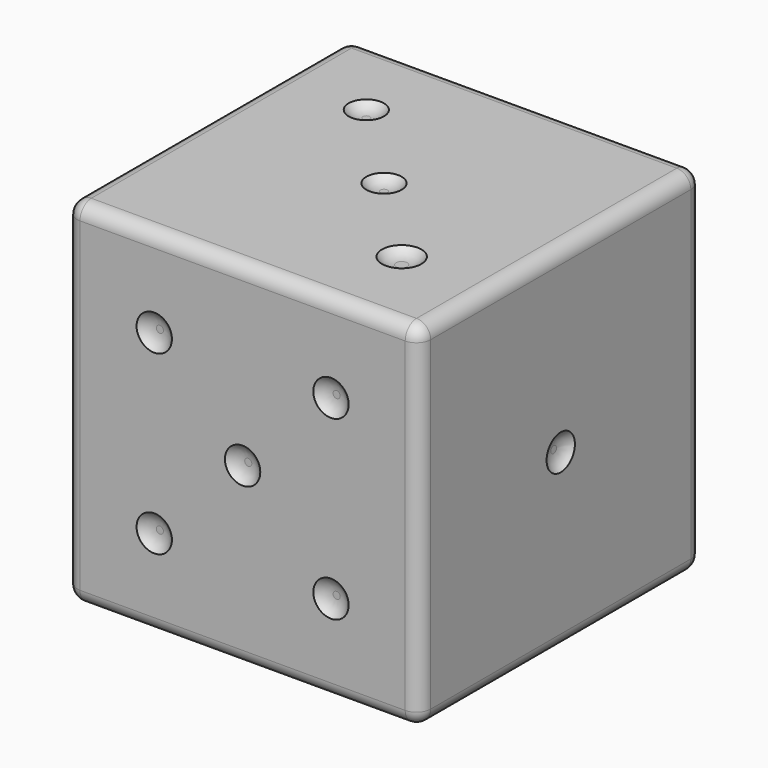
from build123d import *

# Parameters (mm, degrees)
F0_W      = 50
F0_H      = 50
F1_DEPTH  = 50
F3_R      = 2.5
F6_DEPTH  = 1
F5_R      = 2.5
F7_DEPTH  = 1
F2_R      = 2.786439664
F2_R_2    = 2.5
F8_DEPTH  = 1
F9_R      = 2.5
F10_DEPTH = 1
F4_R      = 2.5
F11_DEPTH = 1
F12_R     = 2.5
F13_DEPTH = 1
F16_W     = 40
F16_H     = 40
F17_DEPTH = 30
F18_DEPTH = 30
F19_R     = 2


# Not quite as in the source:
# - a fillet or chamfer that OpenCascade refuses, or shapes differently, is made with other operations: its cross-section is extruded or revolved along the edge and cut away or added


with BuildPart() as f1:
    # F0 (on Top) → F1 (new body)
    with BuildSketch(Plane.XY):
        Rectangle(F0_W, F0_H)
    extrude(amount=F1_DEPTH)

    # F3 (on face) → F6 (cut)
    with BuildSketch(Plane(origin=(-25, 0, 0), x_dir=(0, -1, 0), z_dir=(-1, 0, 0))):
        with Locations((0, 37.5)):
            Circle(F3_R)
        with Locations((12.5, 37.5)):
            Circle(F3_R)
        with Locations((12.5, 12.5)):
            Circle(F3_R)
        with Locations((0, 12.5)):
            Circle(F3_R)
        with Locations((-12.5, 12.5)):
            Circle(F3_R)
        with Locations((-12.5, 37.5)):
            Circle(F3_R)
    extrude(amount=-F6_DEPTH, mode=Mode.SUBTRACT)

    # F5 (on face) → F7 (cut)
    with BuildSketch(Plane.YZ.offset(25)):
        with Locations((0, 24.6321298182)):
            Circle(F5_R)
    extrude(amount=-F7_DEPTH, mode=Mode.SUBTRACT)

    # F2 (on face) → F8 (cut)
    with BuildSketch(Plane.XY.offset(50)):
        with Locations((12.5, -12.5)):
            Circle(F2_R)
        Circle(F2_R_2)
        with Locations((-12.5, 12.5)):
            Circle(F2_R_2)
    extrude(amount=-F8_DEPTH, mode=Mode.SUBTRACT)

    # F9 (on face) → F10 (cut)
    with BuildSketch(Plane(origin=(0, 0, 0), x_dir=(1, 0, 0), z_dir=(0, 0, -1))):
        with Locations((12.5, 12.5)):
            Circle(F9_R)
        with Locations((12.5, -12.5)):
            Circle(F9_R)
        with Locations((-12.5, -12.5)):
            Circle(F9_R)
        with Locations((-12.5, 12.5)):
            Circle(F9_R)
    extrude(amount=-F10_DEPTH, mode=Mode.SUBTRACT)

    # F4 (on face) → F11 (cut)
    with BuildSketch(Plane.XZ.offset(25)):
        with Locations((-12.5, 37.5)):
            Circle(F4_R)
        with Locations((12.5, 12.5)):
            Circle(F4_R)
        with Locations((12.5, 37.5)):
            Circle(F4_R)
        with Locations((0, 25)):
            Circle(F4_R)
        with Locations((-12.5, 12.5)):
            Circle(F4_R)
    extrude(amount=-F11_DEPTH, mode=Mode.SUBTRACT)

    # F12 (on face) → F13 (cut)
    with BuildSketch(Plane(origin=(0, 25, 0), x_dir=(-1, 0, 0), z_dir=(0, 1, 0))):
        with Locations((-12.5, 37.5)):
            Circle(F12_R)
        with Locations((12.5, 12.5)):
            Circle(F12_R)
    extrude(amount=-F13_DEPTH, mode=Mode.SUBTRACT)

    # F16 (on line) → F17 (cut)
    with BuildSketch(Plane(origin=(7.3781074025, 0, 0), x_dir=(0, -1, 0), z_dir=(-1, 0, 0))):
        with Locations((0, 25)):
            Rectangle(F16_W, F16_H)
    extrude(amount=F17_DEPTH, mode=Mode.SUBTRACT)

    # F19
    f19_edges = [f1.edges().sort_by_distance(p)[0] for p in [
        (-25, 0, 50),
        (-25, 25, 25),
        (-25, 0, 0),
        (-25, -25, 25),
        (0, -25, 50),
        (25, 0, 50),
        (0, 25, 50),
        (0, -25, 0),
        (25, 0, 0),
        (0, 25, 0),
        (25, 25, 25),
        (25, -25, 25),
    ]]
    fillet(f19_edges, radius=F19_R)

    # F20: fillet of radius 2.5 on 21 edges, made by hand

    # F20_s1 → F20_t2 (revolve)
    with BuildSketch(Plane.XZ.offset(-12.5)):
        with BuildLine():
            ThreePointArc((-10, 50), (-10.8819660113, 49.2639320225), (-12, 49))
            Line((-12, 49), (-10, 49))
            Line((-10, 49), (-10, 50))
        make_face()
    revolve(axis=Axis((-12.5, 12.5, 49), (0, 0, 1)))

    # F20_s3 → F20_t4 (revolve)
    with BuildSketch(Plane.XZ.offset(12.5)):
        with BuildLine():
            ThreePointArc((15.286439664, 50), (14.4044736528, 49.2639320225), (13.286439664, 49))
            Line((13.286439664, 49), (15.286439664, 49))
            Line((15.286439664, 49), (15.286439664, 50))
        make_face()
    revolve(axis=Axis((12.5, -12.5, 49), (0, 0, 1)))

    # F20_s5 → F20_t6 (revolve)
    with BuildSketch(Plane.XZ):
        with BuildLine():
            ThreePointArc((2.5, 50), (1.6180339887, 49.2639320225), (0.5, 49))
            Line((0.5, 49), (2.5, 49))
            Line((2.5, 49), (2.5, 50))
        make_face()
    revolve(axis=Axis((0, 0, 49), (0, 0, 1)))

    # F20_s7 → F20_t8 (revolve)
    with BuildSketch(Plane.XY.offset(37.5)):
        with BuildLine():
            ThreePointArc((10, 25), (10.8819660113, 24.2639320225), (12, 24))
            Line((12, 24), (10, 24))
            Line((10, 24), (10, 25))
        make_face()
    revolve(axis=Axis((12.5, 24, 37.5), (0, 1, 0)))

    # F20_s9 → F20_t10 (revolve)
    with BuildSketch(Plane.XY.offset(12.5)):
        with BuildLine():
            ThreePointArc((-15, 25), (-14.1180339887, 24.2639320225), (-13, 24))
            Line((-13, 24), (-15, 24))
            Line((-15, 24), (-15, 25))
        make_face()
    revolve(axis=Axis((-12.5, 24, 12.5), (0, 1, 0)))

    # F20_s11 → F20_t12 (revolve)
    with BuildSketch(Plane.XY.offset(37.5)):
        with BuildLine():
            ThreePointArc((-25, 10), (-24.2639320225, 10.8819660113), (-24, 12))
            Line((-24, 12), (-24, 10))
            Line((-24, 10), (-25, 10))
        make_face()
    revolve(axis=Axis((-24, 12.5, 37.5), (-1, 0, 0)))

    # F20_s13 → F20_t14 (revolve)
    with BuildSketch(Plane.XY.offset(12.5)):
        with BuildLine():
            ThreePointArc((-25, -2.5), (-24.2639320225, -1.6180339887), (-24, -0.5))
            Line((-24, -0.5), (-24, -2.5))
            Line((-24, -2.5), (-25, -2.5))
        make_face()
    revolve(axis=Axis((-24, 0, 12.5), (-1, 0, 0)))

    # F20_s15 → F20_t16 (revolve)
    with BuildSketch(Plane.XY.offset(12.5)):
        with BuildLine():
            ThreePointArc((-25, 10), (-24.2639320225, 10.8819660113), (-24, 12))
            Line((-24, 12), (-24, 10))
            Line((-24, 10), (-25, 10))
        make_face()
    revolve(axis=Axis((-24, 12.5, 12.5), (-1, 0, 0)))

    # F20_s17 → F20_t18 (revolve)
    with BuildSketch(Plane.XY.offset(37.5)):
        with BuildLine():
            ThreePointArc((-25, -2.5), (-24.2639320225, -1.6180339887), (-24, -0.5))
            Line((-24, -0.5), (-24, -2.5))
            Line((-24, -2.5), (-25, -2.5))
        make_face()
    revolve(axis=Axis((-24, 0, 37.5), (-1, 0, 0)))

    # F20_s19 → F20_t20 (revolve)
    with BuildSketch(Plane.XY.offset(37.5)):
        with BuildLine():
            ThreePointArc((-25, -15), (-24.2639320225, -14.1180339887), (-24, -13))
            Line((-24, -13), (-24, -15))
            Line((-24, -15), (-25, -15))
        make_face()
    revolve(axis=Axis((-24, -12.5, 37.5), (-1, 0, 0)))

    # F20_s21 → F20_t22 (revolve)
    with BuildSketch(Plane.XY.offset(12.5)):
        with BuildLine():
            ThreePointArc((-25, -15), (-24.2639320225, -14.1180339887), (-24, -13))
            Line((-24, -13), (-24, -15))
            Line((-24, -15), (-25, -15))
        make_face()
    revolve(axis=Axis((-24, -12.5, 12.5), (-1, 0, 0)))

    # F20_s23 → F20_t24 (revolve)
    with BuildSketch(Plane.XZ.offset(12.5)):
        with BuildLine():
            ThreePointArc((15, 0), (14.1180339887, 0.7360679775), (13, 1))
            Line((13, 1), (15, 1))
            Line((15, 1), (15, 0))
        make_face()
    revolve(axis=Axis((12.5, -12.5, 1), (0, 0, -1)))

    # F20_s25 → F20_t26 (revolve)
    with BuildSketch(Plane.XZ.offset(-12.5)):
        with BuildLine():
            ThreePointArc((15, 0), (14.1180339887, 0.7360679775), (13, 1))
            Line((13, 1), (15, 1))
            Line((15, 1), (15, 0))
        make_face()
    revolve(axis=Axis((12.5, 12.5, 1), (0, 0, -1)))

    # F20_s27 → F20_t28 (revolve)
    with BuildSketch(Plane.XY.offset(12.5)):
        with BuildLine():
            ThreePointArc((-10, -25), (-10.8819660113, -24.2639320225), (-12, -24))
            Line((-12, -24), (-10, -24))
            Line((-10, -24), (-10, -25))
        make_face()
    revolve(axis=Axis((-12.5, -24, 12.5), (0, -1, 0)))

    # F20_s29 → F20_t30 (revolve)
    with BuildSketch(Plane.XZ.offset(12.5)):
        with BuildLine():
            ThreePointArc((-10, 0), (-10.8819660113, 0.7360679775), (-12, 1))
            Line((-12, 1), (-10, 1))
            Line((-10, 1), (-10, 0))
        make_face()
    revolve(axis=Axis((-12.5, -12.5, 1), (0, 0, -1)))

    # F20_s31 → F20_t32 (revolve)
    with BuildSketch(Plane.XZ.offset(-12.5)):
        with BuildLine():
            ThreePointArc((-10, 0), (-10.8819660113, 0.7360679775), (-12, 1))
            Line((-12, 1), (-10, 1))
            Line((-10, 1), (-10, 0))
        make_face()
    revolve(axis=Axis((-12.5, 12.5, 1), (0, 0, -1)))

    # F20_s33 → F20_t34 (revolve)
    with BuildSketch(Plane.XY.offset(24.6321298182)):
        with BuildLine():
            ThreePointArc((25, 2.5), (24.2639320225, 1.6180339887), (24, 0.5))
            Line((24, 0.5), (24, 2.5))
            Line((24, 2.5), (25, 2.5))
        make_face()
    revolve(axis=Axis((24, 0, 24.6321298182), (1, 0, 0)))

    # F20_s35 → F20_t36 (revolve)
    with BuildSketch(Plane.XY.offset(25)):
        with BuildLine():
            ThreePointArc((2.5, -25), (1.6180339887, -24.2639320225), (0.5, -24))
            Line((0.5, -24), (2.5, -24))
            Line((2.5, -24), (2.5, -25))
        make_face()
    revolve(axis=Axis((0, -24, 25), (0, -1, 0)))

    # F20_s37 → F20_t38 (revolve)
    with BuildSketch(Plane.XY.offset(12.5)):
        with BuildLine():
            ThreePointArc((15, -25), (14.1180339887, -24.2639320225), (13, -24))
            Line((13, -24), (15, -24))
            Line((15, -24), (15, -25))
        make_face()
    revolve(axis=Axis((12.5, -24, 12.5), (0, -1, 0)))

    # F20_s39 → F20_t40 (revolve)
    with BuildSketch(Plane.XY.offset(37.5)):
        with BuildLine():
            ThreePointArc((15, -25), (14.1180339887, -24.2639320225), (13, -24))
            Line((13, -24), (15, -24))
            Line((15, -24), (15, -25))
        make_face()
    revolve(axis=Axis((12.5, -24, 37.5), (0, -1, 0)))

    # F20_s41 → F20_t42 (revolve)
    with BuildSketch(Plane.XY.offset(37.5)):
        with BuildLine():
            ThreePointArc((-10, -25), (-10.8819660113, -24.2639320225), (-12, -24))
            Line((-12, -24), (-10, -24))
            Line((-10, -24), (-10, -25))
        make_face()
    revolve(axis=Axis((-12.5, -24, 37.5), (0, -1, 0)))


with BuildPart() as f18:
    # F16 (on line) → F18 (new body)
    with BuildSketch(Plane(origin=(7.3781074025, 0, 0), x_dir=(0, -1, 0), z_dir=(-1, 0, 0))):
        with Locations((0, 25)):
            Rectangle(F16_W, F16_H)
    extrude(amount=F18_DEPTH)


solid = Compound([f1.part, f18.part])
